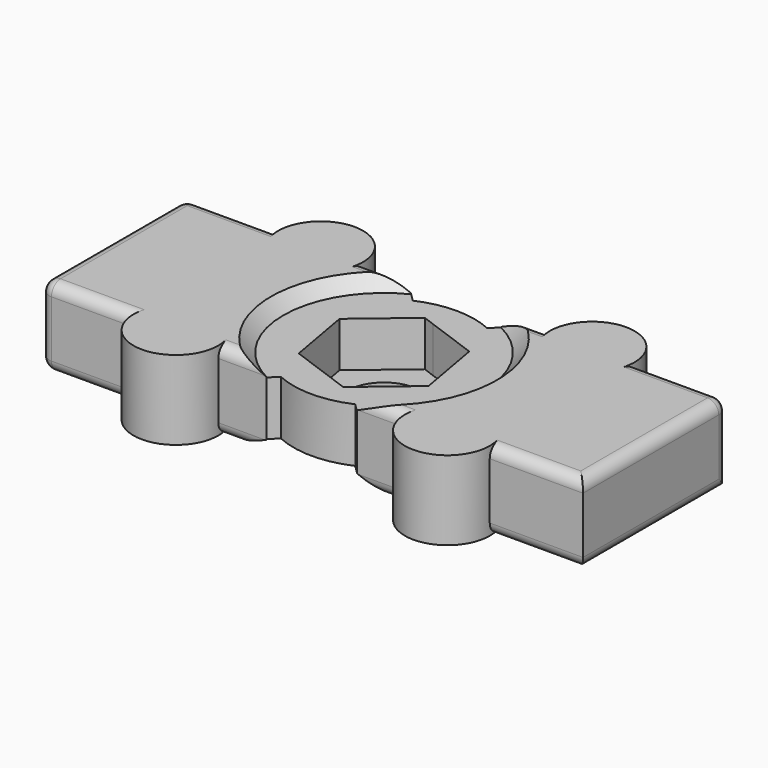
from build123d import *

# Parameters (mm, degrees)
F1_DEPTH     = 3.048
F2_DEPTH     = 4.445
F3_T4_ANGLE  = 205.1460272103
F3_T9_ANGLE  = 205.1460272103
F3_T14_ANGLE = 205.1460272103
F3_T19_ANGLE = 205.1460272103
F4_R         = 1.27
F5_R         = 4.064
F6_DEPTH     = 1.016


# Not quite as in the source:
# - a fillet or chamfer that OpenCascade refuses, or shapes differently, is made with other operations: its cross-section is extruded or revolved along the edge and cut away or added


with BuildPart() as f1:
    # F0 (on Top) → F1 (new body, symmetric)
    with BuildSketch(Plane.XY):
        with BuildLine():
            ThreePointArc((4.1802083301, 9.2602083301), (2.1379760717, 9.932505138), (0, 10.16))
            ThreePointArc((0, 10.16), (-2.1379760717, 9.932505138), (-4.1802083301, 9.2602083301))
            ThreePointArc((-4.1802083301, 9.2602083301), (-10.16, 0), (-4.1802083301, -9.2602083301))
            ThreePointArc((-4.1802083301, -9.2602083301), (0, -10.16), (4.1802083301, -9.2602083301))
            ThreePointArc((4.1802083301, -9.2602083301), (8.5351191156, -5.511564359), (10.16, 0))
            ThreePointArc((10.16, 0), (8.5351191156, 5.511564359), (4.1802083301, 9.2602083301))
        make_face()
        Polygon((-5.7207672085, -4.8174884064), (-7.0324509466, 2.5455855286), (-1.3116837381, 7.3630739349), (0, 6.8882745845), (5.7207672085, 4.8174884064), (7.0324509466, -2.5455855286), (4.5967240587, -4.5967240587), (1.3116837381, -7.3630739349), (0, -6.8882745845), align=None, mode=Mode.SUBTRACT)
    extrude(amount=F1_DEPTH, both=True)

    # F0 (on Top) → F2 (join, symmetric)
    with BuildSketch(Plane.XY):
        with BuildLine():
            ThreePointArc((-4.1802083301, -9.2602083301), (-10.16, 0), (-4.1802083301, 9.2602083301))
            Line((-4.1802083301, 9.2602083301), (-5.08, 10.16))
            Line((-5.08, 10.16), (-10.4775, 10.16))
            ThreePointArc((-10.4775, 10.16), (-15.24, 14.9225), (-20.0025, 10.16))
            Line((-20.0025, 10.16), (-30.48, 10.16))
            Line((-30.48, 10.16), (-30.48, -10.16))
            Line((-30.48, -10.16), (-20.0025, -10.16))
            ThreePointArc((-20.0025, -10.16), (-15.24, -14.9225), (-10.4775, -10.16))
            Line((-10.4775, -10.16), (-5.08, -10.16))
            Line((-5.08, -10.16), (-4.1802083301, -9.2602083301))
        make_face()
        with BuildLine():
            Line((5.08, 10.16), (4.1802083301, 9.2602083301))
            ThreePointArc((4.1802083301, 9.2602083301), (8.5351191156, 5.511564359), (10.16, 0))
            ThreePointArc((10.16, 0), (8.5351191156, -5.511564359), (4.1802083301, -9.2602083301))
            Line((4.1802083301, -9.2602083301), (5.08, -10.16))
            Line((5.08, -10.16), (10.4775, -10.16))
            ThreePointArc((10.4775, -10.16), (15.24, -14.9225), (20.0025, -10.16))
            Line((20.0025, -10.16), (30.48, -10.16))
            Line((30.48, -10.16), (30.48, 10.16))
            Line((30.48, 10.16), (20.0025, 10.16))
            ThreePointArc((20.0025, 10.16), (15.24, 14.9225), (10.4775, 10.16))
            Line((10.4775, 10.16), (5.08, 10.16))
        make_face()
    extrude(amount=F2_DEPTH, both=True)

    # F3: chamfer of 2.54 on 4 edges, made by hand


with BuildPart() as f3_tool2:
    # F3_s3 → F3_t4 (revolve)
    with BuildSketch(Plane(origin=(0, 0, 0), x_dir=(0, 0, 1), z_dir=(0.9760193995, 0.217683559, 0))):
        Polygon((4.445, 12.7), (1.905, 10.16), (4.445, 10.16), align=None)
    revolve(axis=Axis((0, 0, 4.445), (0, 0, -1)), revolution_arc=F3_T4_ANGLE)

    split(bisect_by=Plane.XY.offset(3.048), keep=Keep.TOP)


with BuildPart() as f1_1:
    add(f1.part)

    # F3_t1: cut F3_tool2
    add(f3_tool2.part, mode=Mode.SUBTRACT)


with BuildPart() as f3_tool7:
    # F3_s8 → F3_t9 (revolve)
    with BuildSketch(Plane(origin=(0, 0, 0), x_dir=(0, 0, 1), z_dir=(-0.9760193995, -0.217683559, 0))):
        Polygon((1.905, 10.16), (4.445, 12.7), (4.445, 10.16), align=None)
    revolve(axis=Axis((0, 0, 4.445), (0, 0, -1)), revolution_arc=F3_T9_ANGLE)

    split(bisect_by=Plane.XY.offset(3.048), keep=Keep.TOP)


with BuildPart() as f1_2:
    add(f1_1.part)

    # F3_t6: cut F3_tool7
    add(f3_tool7.part, mode=Mode.SUBTRACT)


with BuildPart() as f3_tool12:
    # F3_s13 → F3_t14 (revolve)
    with BuildSketch(Plane(origin=(0, 0, 0), x_dir=(0, 0, 1), z_dir=(-0.9760193995, -0.217683559, 0))):
        Polygon((-4.445, 12.7), (-1.905, 10.16), (-4.445, 10.16), align=None)
    revolve(axis=Axis((0, 0, -4.445), (0, 0, -1)), revolution_arc=F3_T14_ANGLE)

    split(bisect_by=Plane.XY.offset(-3.048), keep=Keep.BOTTOM)


with BuildPart() as f1_3:
    add(f1_2.part)

    # F3_t11: cut F3_tool12
    add(f3_tool12.part, mode=Mode.SUBTRACT)


with BuildPart() as f3_tool17:
    # F3_s18 → F3_t19 (revolve)
    with BuildSketch(Plane(origin=(0, 0, 0), x_dir=(0, 0, 1), z_dir=(0.9760193995, 0.217683559, 0))):
        Polygon((-1.905, 10.16), (-4.445, 12.7), (-4.445, 10.16), align=None)
    revolve(axis=Axis((0, 0, -4.445), (0, 0, -1)), revolution_arc=F3_T19_ANGLE)

    split(bisect_by=Plane.XY.offset(-3.048), keep=Keep.BOTTOM)


with BuildPart() as f1_4:
    add(f1_3.part)

    # F3_t16: cut F3_tool17
    add(f3_tool17.part, mode=Mode.SUBTRACT)

    # F4
    f4_edges = [f1_4.edges().sort_by_distance(p)[0] for p in [
        (-25.24125, -10.16, 4.445),
        (-30.48, 0, 4.445),
        (-25.24125, 10.16, 4.445),
        (25.24125, -10.16, 4.445),
        (30.48, 0, 4.445),
        (25.24125, 10.16, 4.445),
        (-25.24125, -10.16, -4.445),
        (-30.48, -10.16, 0),
        (25.24125, -10.16, -4.445),
        (30.48, 0, -4.445),
        (30.48, 10.16, 0),
        (-30.48, 10.16, 0),
        (-25.24125, 10.16, -4.445),
        (-30.48, 0, -4.445),
        (-9.04875, 10.16, 4.445),
        (9.04875, 10.16, 4.445),
        (-9.04875, -10.16, 4.445),
        (9.04875, -10.16, 4.445),
        (9.04875, 10.16, -4.445),
        (-9.04875, 10.16, -4.445),
        (-9.04875, -10.16, -4.445),
        (9.04875, -10.16, -4.445),
    ]]
    fillet(f4_edges, radius=F4_R)

    # F5 (on face) → F6 (join)
    with BuildSketch(Plane(origin=(0, 0, -3.048), x_dir=(1, 0, 0), z_dir=(0, 0, -1))):
        with BuildLine():
            ThreePointArc((4.4189755144, -9.4989755144), (8.8332738002, -5.6330413093), (10.4765395251, 0))
            ThreePointArc((10.4765395251, 0), (8.8332738002, 5.6330413093), (4.4189755144, 9.4989755144))
            Line((4.4189755144, 9.4989755144), (4.1802083301, 9.2602083301))
            ThreePointArc((4.1802083301, 9.2602083301), (0, 10.16), (-4.1802083301, 9.2602083301))
            Line((-4.1802083301, 9.2602083301), (-4.4189755144, 9.4989755144))
            ThreePointArc((-4.4189755144, 9.4989755144), (-10.4765395251, 0), (-4.4189755144, -9.4989755144))
            Line((-4.4189755144, -9.4989755144), (-4.1802083301, -9.2602083301))
            ThreePointArc((-4.1802083301, -9.2602083301), (0, -10.16), (4.1802083301, -9.2602083301))
            Line((4.1802083301, -9.2602083301), (4.4189755144, -9.4989755144))
        make_face()
        Polygon((-1.3116837381, -7.3630739349), (-7.0324509466, -2.5455855286), (-5.7207672085, 4.8174884064), (1.3116837381, 7.3630739349), (7.0324509466, 2.5455855286), (5.7207672085, -4.8174884064), align=None, mode=Mode.SUBTRACT)
        Polygon((-5.7207672085, 4.8174884064), (-7.0324509466, -2.5455855286), (-1.3116837381, -7.3630739349), (5.7207672085, -4.8174884064), (7.0324509466, 2.5455855286), (1.3116837381, 7.3630739349), align=None)
        Circle(F5_R, mode=Mode.SUBTRACT)
    extrude(amount=-F6_DEPTH)


solid = f1_4.part
